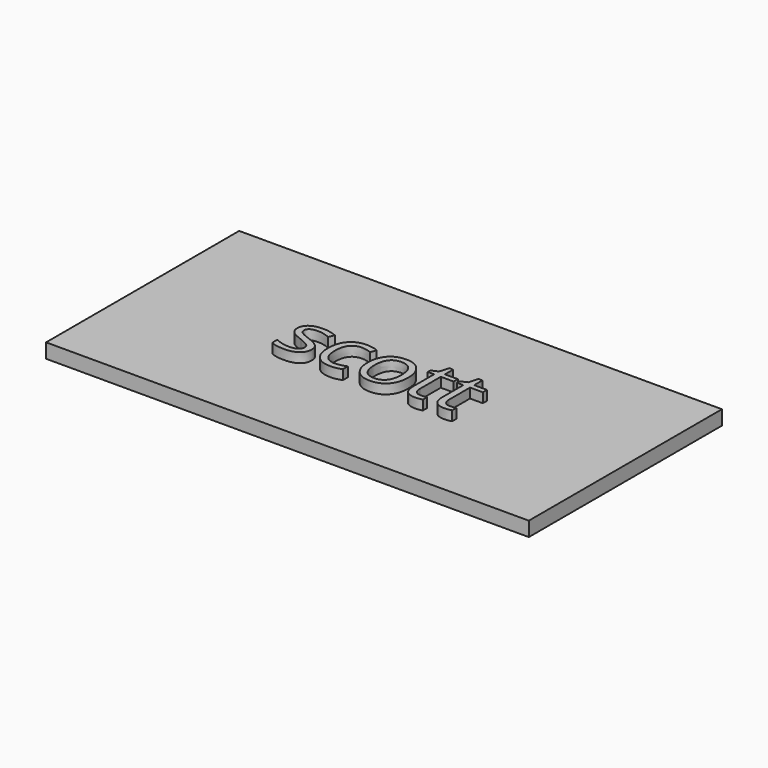
from build123d import *

# Parameters (mm, degrees)
F0_W         = 100
F0_H         = 50
F1_DEPTH     = 3
F2_TEXT_SIZE = 17.1431805938
F3_DEPTH     = 2


# Not quite as in the source:
# - Text() gives the source's letters only with a copy of the font that has no kerning and outlines rounded to 1/6400 em; it was checked with that copy


with BuildPart() as f1:
    # F0 (on Top) → F1 (new body)
    with BuildSketch(Plane.XY):
        with Locations((50, 25)):
            Rectangle(F0_W, F0_H)
    extrude(amount=F1_DEPTH)

    # F2 (on face) → F3 (join)
    with BuildSketch(Plane.XY.offset(3)):
        with Locations((30.130833853, 19.3748865277)):
            Text('scott', F2_TEXT_SIZE, font='Open Sans', text_align=(TextAlign.LEFT, TextAlign.BOTTOM))
    extrude(amount=F3_DEPTH)


solid = f1.part
